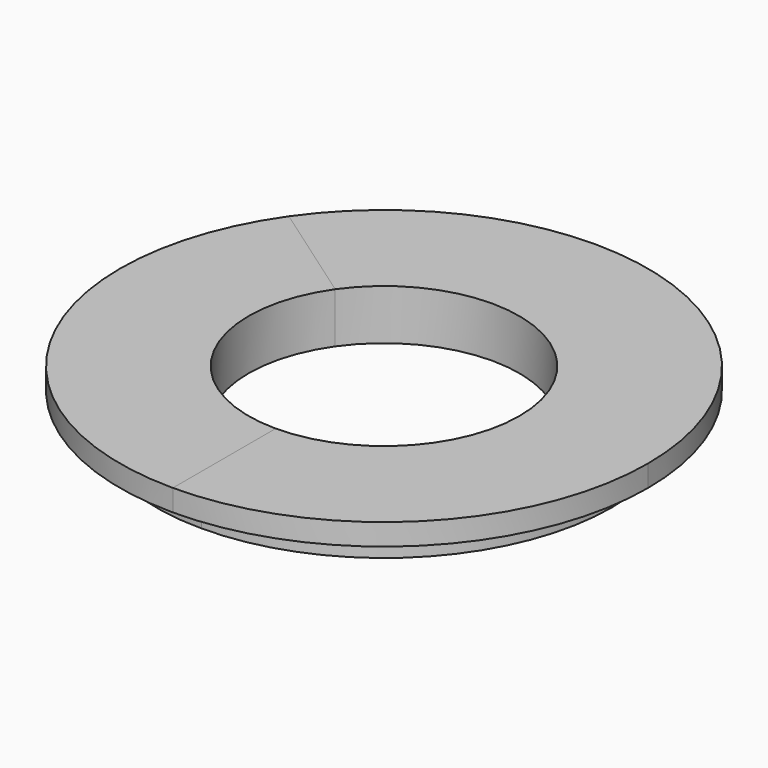
from build123d import *

# Parameters (mm, degrees)
F1_DEPTH = 3
F2_DEPTH = 4
F3_DEPTH = 3
F4_DEPTH = 4


with BuildPart() as f1:
    # F0 (on Top) → F1 (new body)
    with BuildSketch(Plane.XY):
        with BuildLine():
            Line((-30.0628800254, 21.0502552141), (-25.967119804, 18.1823730323))
            ThreePointArc((-25.967119804, 18.1823730323), (9.5323738443, 30.2328273387), (31.7, 0))
            ThreePointArc((31.7, 0), (22.4152849636, -22.4152849636), (0, -31.7))
            Line((0, -31.7), (0, -36.7))
            ThreePointArc((0, -36.7), (25.9508188695, -25.9508188695), (36.7, 0))
            ThreePointArc((36.7, 0), (11.0359028418, 35.0014120925), (-30.0628800254, 21.0502552141))
        make_face()
        with BuildLine():
            ThreePointArc((-15.4205372337, 10.7975764143), (5.6607866757, 17.9537215978), (18.825, 0))
            ThreePointArc((18.825, 0), (13.3112851558, -13.3112851558), (0, -18.825))
            Line((0, -18.825), (0, -31.7))
            ThreePointArc((0, -31.7), (22.4152849636, -22.4152849636), (31.7, 0))
            ThreePointArc((31.7, 0), (9.5323738443, 30.2328273387), (-25.967119804, 18.1823730323))
            Line((-25.967119804, 18.1823730323), (-15.4205372337, 10.7975764143))
        make_face()
    extrude(amount=F1_DEPTH)

    # F0 (on Top) → F2 (join)
    with BuildSketch(Plane.XY):
        with BuildLine():
            ThreePointArc((-15.4205372337, 10.7975764143), (5.6607866757, 17.9537215978), (18.825, 0))
            ThreePointArc((18.825, 0), (13.3112851558, -13.3112851558), (0, -18.825))
            Line((0, -18.825), (0, -31.7))
            ThreePointArc((0, -31.7), (22.4152849636, -22.4152849636), (31.7, 0))
            ThreePointArc((31.7, 0), (9.5323738443, 30.2328273387), (-25.967119804, 18.1823730323))
            Line((-25.967119804, 18.1823730323), (-15.4205372337, 10.7975764143))
        make_face()
    extrude(amount=-F2_DEPTH)


with BuildPart() as f3:
    # F0 (on Top) → F3 (new body)
    with BuildSketch(Plane.XY):
        with BuildLine():
            ThreePointArc((0, -18.825), (-16.6979789346, -8.6924176441), (-15.4205372337, 10.7975764143))
            Line((-15.4205372337, 10.7975764143), (-25.967119804, 18.1823730323))
            ThreePointArc((-25.967119804, 18.1823730323), (-28.1182434117, -14.6374310396), (0, -31.7))
            Line((0, -31.7), (0, -18.825))
        make_face()
        with BuildLine():
            ThreePointArc((0, -31.7), (-28.1182434117, -14.6374310396), (-25.967119804, 18.1823730323))
            Line((-25.967119804, 18.1823730323), (-30.0628800254, 21.0502552141))
            ThreePointArc((-30.0628800254, 21.0502552141), (-32.5532975776, -16.9461741057), (0, -36.7))
            Line((0, -36.7), (0, -31.7))
        make_face()
    extrude(amount=F3_DEPTH)

    # F0 (on Top) → F4 (join)
    with BuildSketch(Plane.XY):
        with BuildLine():
            ThreePointArc((0, -18.825), (-16.6979789346, -8.6924176441), (-15.4205372337, 10.7975764143))
            Line((-15.4205372337, 10.7975764143), (-25.967119804, 18.1823730323))
            ThreePointArc((-25.967119804, 18.1823730323), (-28.1182434117, -14.6374310396), (0, -31.7))
            Line((0, -31.7), (0, -18.825))
        make_face()
    extrude(amount=-F4_DEPTH)


solid = Compound([f1.part, f3.part])
